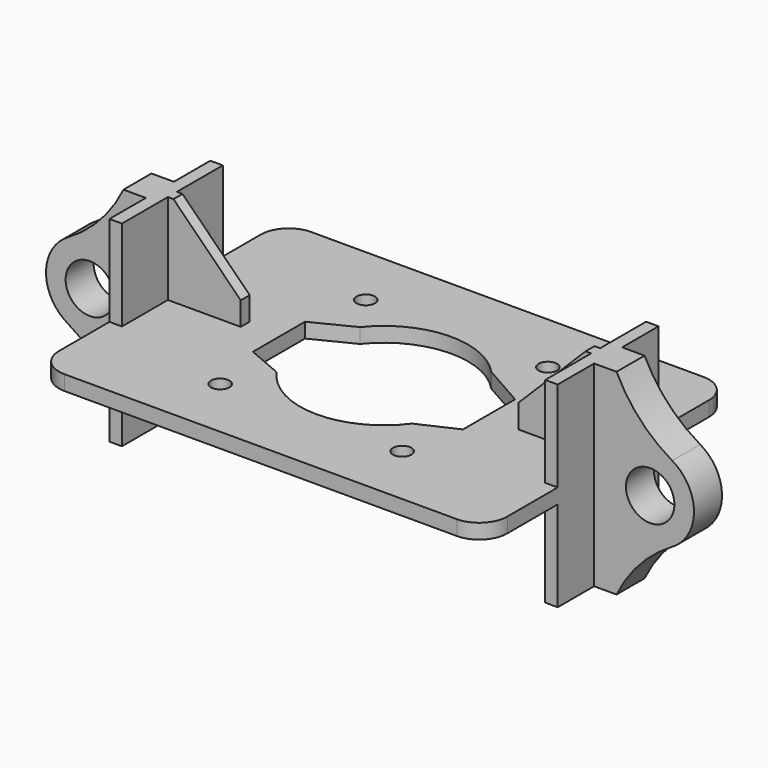
from build123d import *

# Parameters (mm, degrees)
F0_R      = 8.382
F1_DEPTH  = 6.731
F2_W      = 114.3
F2_H      = 177.8
F3_DEPTH  = 11.3284
F4_R      = 21.971
F5_DEPTH  = 15.875
F6_W      = 66.04
F6_H      = 10.16
F7_DEPTH  = 177.8
F8_SIZE   = 60.96
F10_DEPTH = 95.632


# Not quite as in the source:
# - a pattern or mirror of a feature is missing from the dataset's text; its kind, count and spacing are read off the source's solid


with BuildPart() as f1:
    # F0 (on Top) → F1 (new body, symmetric)
    with BuildSketch(Plane.XY):
        with BuildLine():
            Line((177.8, 139.7), (-177.8, 139.7))
            ThreePointArc((-177.8, 139.7), (-195.7605122421, 132.2605122421), (-203.2, 114.3))
            Line((-203.2, 114.3), (-203.2, -114.3))
            ThreePointArc((-203.2, -114.3), (-195.7605122421, -132.2605122421), (-177.8, -139.7))
            Line((-177.8, -139.7), (177.8, -139.7))
            ThreePointArc((177.8, -139.7), (195.7605122421, -132.2605122421), (203.2, -114.3))
            Line((203.2, -114.3), (203.2, 114.3))
            ThreePointArc((203.2, 114.3), (195.7605122421, 132.2605122421), (177.8, 139.7))
        make_face()
        with Locations((-82.55, -82.55)):
            Circle(F0_R, mode=Mode.SUBTRACT)
        with Locations((82.55, -82.55)):
            Circle(F0_R, mode=Mode.SUBTRACT)
        with Locations((-82.55, 82.55)):
            Circle(F0_R, mode=Mode.SUBTRACT)
        with Locations((82.55, 82.55)):
            Circle(F0_R, mode=Mode.SUBTRACT)
    extrude(amount=F1_DEPTH, both=True)

    # F2 (on face) → F3 (join)
    with BuildSketch(Plane(origin=(-203.2, 0, 0), x_dir=(0, -1, 0), z_dir=(-1, 0, 0))):
        Rectangle(F2_W, F2_H)
    f3 = extrude(amount=-F3_DEPTH)

    # F3_copies: F3 across plane
    add(f3.mirror(Plane(origin=(0, 0, 0), x_dir=(0, 0, 1), z_dir=(1, 0, 0))))

    # F4 (on Front) → F5 (join, symmetric)
    with BuildSketch(Plane.XZ):
        with BuildLine():
            ThreePointArc((-223.52, 88.9), (-244.6799408534, 57.8520750061), (-273.9982965787, 34.354186571))
            ThreePointArc((-273.9982965787, 34.354186571), (-293.751, 0), (-273.9982965787, -34.354186571))
            ThreePointArc((-273.9982965787, -34.354186571), (-244.6799408534, -57.8520750061), (-223.52, -88.9))
            Line((-223.52, -88.9), (-203.2, -88.9))
            Line((-203.2, -88.9), (-203.2, -6.731))
            Line((-203.2, -6.731), (-203.2, 6.731))
            Line((-203.2, 6.731), (-203.2, 88.9))
            Line((-203.2, 88.9), (-223.52, 88.9))
        make_face()
        with Locations((-254, 0)):
            Circle(F4_R, mode=Mode.SUBTRACT)
    f5 = extrude(amount=F5_DEPTH, both=True)

    # F5_copies: F5 across plane
    add(f5.mirror(Plane(origin=(0, 0, 0), x_dir=(0, 0, 1), z_dir=(1, 0, 0))))

    # F6 (on face) → F7 (join, through all)
    with BuildSketch(Plane.XY.offset(88.9)):
        with Locations((-158.8516, 0)):
            Rectangle(F6_W, F6_H)
    f7 = extrude(amount=-F7_DEPTH)

    # F7_copies: F7 across plane
    add(f7.mirror(Plane(origin=(0, 0, 0), x_dir=(0, 0, 1), z_dir=(1, 0, 0))))

    # F8
    f8_edges = [f1.edges().sort_by_distance(p)[0] for p in [
        (-125.8316, 0, -88.9),
        (-125.8316, 0, 88.9),
        (125.8316, 0, -88.9),
        (125.8316, 0, 88.9),
    ]]
    chamfer(f8_edges, length=F8_SIZE)

    # F9 (on face) → F10 (cut, through all)
    with BuildSketch(Plane(origin=(0, 0, -6.731), x_dir=(1, 0, 0), z_dir=(0, 0, -1))):
        with BuildLine():
            Line((-95.25, -29.5275), (-59.6566653523, -47.4080402362))
            ThreePointArc((-59.6566653523, -47.4080402362), (-2.9560938308, -76.1426392323), (55.8015879509, -51.8904883592))
            Line((55.8015879509, -51.8904883592), (95.25, -29.5275))
            Line((95.25, -29.5275), (95.25, 29.5275))
            Line((95.25, 29.5275), (61.3953822556, 45.1336574818))
            ThreePointArc((61.3953822556, 45.1336574818), (-1.0966393905, 76.1921083974), (-62.6689060075, 43.3479898015))
            Line((-62.6689060075, 43.3479898015), (-95.25, 29.5275))
            Line((-95.25, 29.5275), (-95.25, -29.5275))
        make_face()
    extrude(amount=-F10_DEPTH, mode=Mode.SUBTRACT)


solid = f1.part
